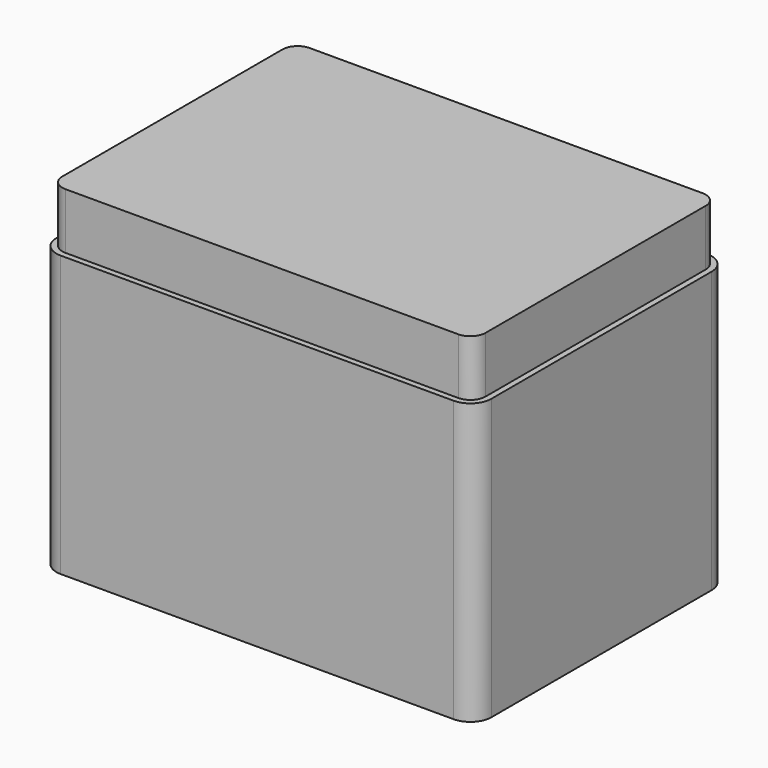
from build123d import *

# Parameters (mm, degrees)
F0_W     = 197.0488578081
F0_H     = 143.7139809132
F1_DEPTH = 76.2
F2_R     = 9.525
F4_DEPTH = 25.4


with BuildPart() as f1:
    # F0 (on Top) → F1 (new body, symmetric)
    with BuildSketch(Plane.XY):
        with Locations((6.136842072, -4.1339993477)):
            Rectangle(F0_W, F0_H)
    extrude(amount=F1_DEPTH, both=True)

    # F2
    f2_edges = [f1.edges().sort_by_distance(p)[0] for p in [
        (-92.387587, -75.99099, 0),
        (-92.387587, 67.722991, 0),
        (104.661271, 67.722991, 0),
        (104.661271, -75.99099, 0),
    ]]
    fillet(f2_edges, radius=F2_R)

    # F3 (on face) → F4 (cut)
    with BuildSketch(Plane.XY.offset(76.2)):
        with BuildLine():
            Line((95.1362709761, 67.7229911089), (-82.862586832, 67.7229911089))
            ThreePointArc((-82.862586832, 67.7229911089), (-89.5977789228, 64.9331831997), (-92.387586832, 58.1979911089))
            Line((-92.387586832, 58.1979911089), (-92.387586832, -66.4659898043))
            ThreePointArc((-92.387586832, -66.4659898043), (-89.5977789228, -73.2011818951), (-82.862586832, -75.9909898043))
            Line((-82.862586832, -75.9909898043), (95.1362709761, -75.9909898043))
            ThreePointArc((95.1362709761, -75.9909898043), (101.8714630669, -73.2011818951), (104.6612709761, -66.4659898043))
            Line((104.6612709761, -66.4659898043), (104.6612709761, 58.1979911089))
            ThreePointArc((104.6612709761, 58.1979911089), (101.8714630669, 64.9331831997), (95.1362709761, 67.7229911089))
        make_face()
        with BuildLine():
            ThreePointArc((-89.720586832, 58.1979911089), (-87.7119251374, 63.0473294143), (-82.862586832, 65.0559911089))
            Line((-82.862586832, 65.0559911089), (95.1362709761, 65.0559911089))
            ThreePointArc((95.1362709761, 65.0559911089), (99.9856092814, 63.0473294143), (101.9942709761, 58.1979911089))
            Line((101.9942709761, 58.1979911089), (101.9942709761, -66.4659898043))
            ThreePointArc((101.9942709761, -66.4659898043), (99.9856092814, -71.3153281096), (95.1362709761, -73.3239898043))
            Line((95.1362709761, -73.3239898043), (-82.862586832, -73.3239898043))
            ThreePointArc((-82.862586832, -73.3239898043), (-87.7119251374, -71.3153281096), (-89.720586832, -66.4659898043))
            Line((-89.720586832, -66.4659898043), (-89.720586832, 58.1979911089))
        make_face(mode=Mode.SUBTRACT)
    extrude(amount=-F4_DEPTH, mode=Mode.SUBTRACT)


solid = f1.part
